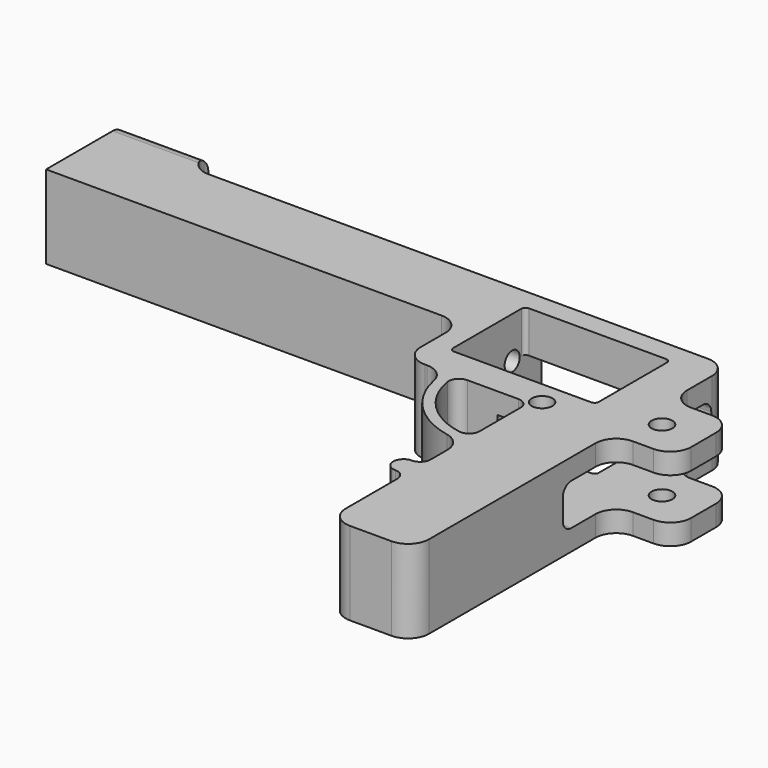
from build123d import *

# Parameters (mm, degrees)
F0_W      = 30
F0_H      = 35
F0_W_2    = 40
F0_H_2    = 12.5
F1_DEPTH  = 20
F2_R      = 4.55
F3_DEPTH  = 300.001
F4_W      = 12.5
F4_H      = 10
F5_DEPTH  = 40.001
F6_R      = 10
F8_DEPTH  = 40.001
F9_R      = 5
F11_DEPTH = 40
F12_W     = 50
F12_H     = 20
F13_DEPTH = 190.001
F14_W     = 70
F14_H     = 45
F15_DEPTH = 40.001
F16_R     = 2
F17_R     = 4.55
F18_DEPTH = 55
F19_R     = 5
F20_R     = 5
F21_DEPTH = 40.0010001
F22_R     = 5
F23_DEPTH = 40.0010001
F25_DEPTH = 20
F26_R     = 4.99999
F27_R     = 7.49999


# Not quite as in the source:
# - a fillet or chamfer is up to 0.001 mm smaller than in the source, because OpenCascade refuses the exact size


with BuildPart() as f1:
    # F0 (on Top) → F1 (new body, symmetric)
    with BuildSketch(Plane.XY):
        Polygon((-60, 0), (-20, 0), (20, 0), (20, 35), (20, 70), (-80, 70), (-80, 35), (-80, 0), align=None)
        Polygon((20, 0), (-20, 0), (-20, -40), (-20, -120), (20, -120), align=None)
        with BuildLine():
            Line((-20, -40), (-20, 0))
            Line((-20, 0), (-60, 0))
            ThreePointArc((-60, 0), (-48.2842712475, -28.2842712475), (-20, -40))
        make_face()
        with Locations((35, 17.5)):
            Rectangle(F0_W, F0_H)
        Polygon((-280, 35), (-80, 35), (-80, 70), (-240, 70), (-280, 70), align=None)
        with Locations((-260, 76.25)):
            Rectangle(F0_W_2, F0_H_2)
    extrude(amount=F1_DEPTH, both=True)

    # F2 (on face) → F3 (cut, through all)
    with BuildSketch(Plane.YZ.offset(20)):
        with Locations((52.5, 0)):
            Circle(F2_R)
    extrude(amount=-F3_DEPTH, mode=Mode.SUBTRACT)

    # F4 (on face) → F5 (cut, through all)
    with BuildSketch(Plane.YZ.offset(-240)):
        with Locations((76.25, 0)):
            Rectangle(F4_W, F4_H)
    extrude(amount=-F5_DEPTH, mode=Mode.SUBTRACT)

    # F6
    f6_edges = [f1.edges().sort_by_distance(p)[0] for p in [
        (-60, 0, 0),
        (-20, -40, 0),
        (-80, 0, 0),
        (-80, 35, 0),
        (20, 0, 0),
        (20, 35, 0),
        (50, 35, 0),
        (50, 0, 0),
        (20, 70, 0),
        (20, -120, 0),
        (-20, -120, 0),
        (-240, 70, 12.5),
        (-240, 70, -12.5),
    ]]
    fillet(f6_edges, radius=F6_R)

    # F7 (on face) → F8 (cut, through all)
    with BuildSketch(Plane(origin=(0, 0, -20), x_dir=(1, 0, 0), z_dir=(0, 0, -1))):
        with BuildLine():
            Line((-20, 0), (-20, 35))
            ThreePointArc((-20, 35), (-44.7487373415, 24.7487373415), (-55, 0))
            Line((-55, 0), (-20, 0))
        make_face()
    extrude(amount=-F8_DEPTH, mode=Mode.SUBTRACT)

    # F9
    f9_edges = [f1.edges().sort_by_distance(p)[0] for p in [
        (-55, 0, 0),
        (-20, -35, 0),
        (-20, 0, 0),
    ]]
    fillet(f9_edges, radius=F9_R)

    # F10 (on face) → F11 (join, through all)
    with BuildSketch(Plane(origin=(0, 0, -20), x_dir=(1, 0, 0), z_dir=(0, 0, -1))):
        with BuildLine():
            ThreePointArc((-25, 63.9897948557), (-21.4644660941, 62.5253287616), (-20, 58.9897948557))
            Line((-20, 58.9897948557), (-20, 78.9897948557))
            ThreePointArc((-20, 78.9897948557), (-21.4644660941, 75.4542609497), (-25, 73.9897948557))
            ThreePointArc((-25, 73.9897948557), (-30, 68.9897948557), (-25, 63.9897948557))
        make_face()
    extrude(amount=-F11_DEPTH)

    # F12 (on face) → F13 (cut, through all)
    with BuildSketch(Plane(origin=(0, 70, 0), x_dir=(-1, 0, 0), z_dir=(0, 1, 0))):
        with Locations((-45, 0)):
            Rectangle(F12_W, F12_H)
    extrude(amount=-F13_DEPTH, mode=Mode.SUBTRACT)

    # F14 (on face) → F15 (cut, through all)
    with BuildSketch(Plane(origin=(0, 0, -20), x_dir=(1, 0, 0), z_dir=(0, 0, -1))):
        with Locations((-35, -37.5)):
            Rectangle(F14_W, F14_H)
    extrude(amount=-F15_DEPTH, mode=Mode.SUBTRACT)

    # F16
    f16_edges = [f1.edges().sort_by_distance(p)[0] for p in [
        (0, 60, 0),
        (0, 15, 0),
        (-70, 60, 0),
        (-70, 15, 0),
    ]]
    fillet(f16_edges, radius=F16_R)

    # F17 (on face) → F18 (cut)
    with BuildSketch(Plane.YZ.offset(20)):
        Polygon((45, 10), (15, 10), (15, -10), (45, -10), (59.5803989155, -10), (59.5803989155, 10), align=None)
        with Locations((52.5, 0)):
            Circle(F17_R, mode=Mode.SUBTRACT)
        Polygon((-10, 10), (-29.5803989155, 10), (-29.5803989155, -10), (-10, -10), (15, -10), (15, 10), align=None)
    extrude(amount=-F18_DEPTH, mode=Mode.SUBTRACT)

    # F19
    f19_edges = [f1.edges().sort_by_distance(p)[0] for p in [
        (0, -29.580399, 10),
        (0, -29.580399, -10),
        (9.61285, 59.580399, 10),
        (9.61285, 59.580399, -10),
    ]]
    fillet(f19_edges, radius=F19_R)

    # F20 (on face) → F21 (cut, through all)
    with BuildSketch(Plane(origin=(0, 0, -20), x_dir=(1, 0, 0), z_dir=(0, 0, -1))):
        with Locations((30, -17.5)):
            Circle(F20_R)
    extrude(amount=-F21_DEPTH, mode=Mode.SUBTRACT)

    # F22 (on face) → F23 (cut, through all)
    with BuildSketch(Plane(origin=(0, 0, -20), x_dir=(1, 0, 0), z_dir=(0, 0, -1))):
        with Locations((-16.4644660941, -3.5355339059)):
            Circle(F22_R)
    extrude(amount=-F23_DEPTH, mode=Mode.SUBTRACT)

    # F24 (on face) → F25 (cut, through all)
    with BuildSketch(Plane(origin=(0, 0, -20), x_dir=(1, 0, 0), z_dir=(0, 0, -1))):
        with BuildLine():
            ThreePointArc((-68, -60), (-69.4142135624, -59.4142135624), (-70, -58))
            Line((-70, -58), (-70, -70))
            Line((-70, -70), (0, -70))
            Line((0, -70), (0, -58))
            ThreePointArc((0, -58), (-0.5857864376, -59.4142135624), (-2, -60))
            Line((-2, -60), (-68, -60))
        make_face()
    extrude(amount=-F25_DEPTH, mode=Mode.SUBTRACT)

    # F26 (radius 5 in the source; OpenCascade refuses exactly that, so slightly less here)
    f26_edges = [f1.edges().sort_by_distance(p)[0] for p in [
        (-255, 70, -5),
        (-255, 70, 5),
    ]]
    fillet(f26_edges, radius=F26_R)

    # F27 (radius 7.5 in the source; OpenCascade refuses exactly that, so slightly less here)
    f27_edges = [f1.edges().sort_by_distance(p)[0] for p in [
        (-260, 82.5, -5),
        (-260, 82.5, -20),
        (-260, 82.5, 5),
        (-260, 82.5, 20),
    ]]
    fillet(f27_edges, radius=F27_R)


solid = f1.part
